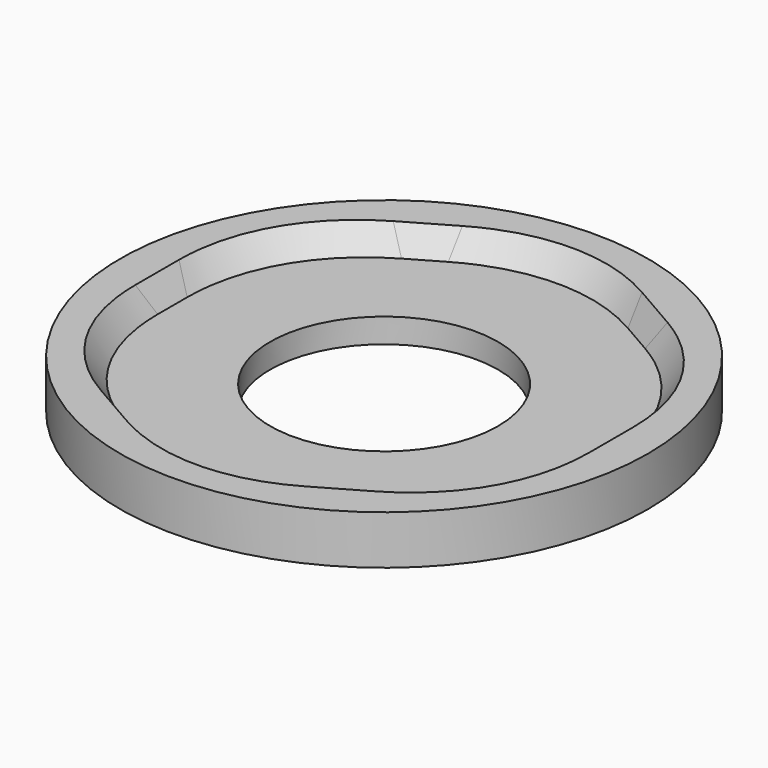
from build123d import *

# Parameters (mm, degrees)
F0_R                   = 32.4
F1_DEPTH               = 6
F0_R_2                 = 14
F2_DEPTH               = 3
F3_DEPTH               = 25
DRAFT_F3_DRAFTED_ANGLE = -32
F4_R                   = 26


# Not quite as in the source:
# - an extrude with a draft is written as a straight extrude whose walls are then drafted


with BuildPart() as f1:
    # F0 (on Top) → F1 (new body)
    with BuildSketch(Plane.XY):
        Circle(F0_R)
        with BuildLine():
            ThreePointArc((25.9807621135, 15), (28.9777747887, 7.7645713531), (30, 0))
            ThreePointArc((30, 0), (28.9777747887, -7.7645713531), (25.9807621135, -15))
            ThreePointArc((25.9807621135, -15), (15, -25.9807621135), (0, -30))
            ThreePointArc((0, -30), (-15, -25.9807621135), (-25.9807621135, -15))
            ThreePointArc((-25.9807621135, -15), (-30, 0), (-25.9807621135, 15))
            ThreePointArc((-25.9807621135, 15), (-15, 25.9807621135), (0, 30))
            ThreePointArc((0, 30), (15, 25.9807621135), (25.9807621135, 15))
        make_face(mode=Mode.SUBTRACT)
        with BuildLine():
            ThreePointArc((0, -30), (15, -25.9807621135), (25.9807621135, -15))
            Line((25.9807621135, -15), (0, -30))
        make_face()
        with BuildLine():
            ThreePointArc((25.9807621135, -15), (28.9777747887, -7.7645713531), (30, 0))
            ThreePointArc((30, 0), (28.9777747887, 7.7645713531), (25.9807621135, 15))
            Line((25.9807621135, 15), (25.9807621135, -15))
        make_face()
        with BuildLine():
            Line((0, 30), (25.9807621135, 15))
            ThreePointArc((25.9807621135, 15), (15, 25.9807621135), (0, 30))
        make_face()
        with BuildLine():
            Line((-25.9807621135, 15), (0, 30))
            ThreePointArc((0, 30), (-15, 25.9807621135), (-25.9807621135, 15))
        make_face()
        with BuildLine():
            Line((-25.9807621135, -15), (-25.9807621135, 15))
            ThreePointArc((-25.9807621135, 15), (-30, 0), (-25.9807621135, -15))
        make_face()
        with BuildLine():
            ThreePointArc((-25.9807621135, -15), (-15, -25.9807621135), (0, -30))
            Line((0, -30), (-25.9807621135, -15))
        make_face()
    extrude(amount=F1_DEPTH)

    # F0 (on Top) → F2 (join)
    with BuildSketch(Plane.XY):
        Polygon((25.9807621135, -15), (25.9807621135, 15), (0, 30), (-25.9807621135, 15), (-25.9807621135, -15), (0, -30), align=None)
        Circle(F0_R_2, mode=Mode.SUBTRACT)
    extrude(amount=F2_DEPTH)


with BuildPart() as f3_drafted:
    # F3 (new): a face of the model
    f3_faces = [f1.part.faces().sort_by_distance(p)[0] for p in [
        (25.1870367202, 0, 3),
    ]]
    extrude(f3_faces, amount=F3_DEPTH)

    # draft_F3_drafted
    draft_f3_drafted_walls = [f3_drafted.faces().sort_by_distance(p)[0] for p in [
        (25.9807621135, 0, 19.6666666667),
        (12.9903810568, 22.5, 19.6666666667),
        (-12.9903810568, 22.5, 19.6666666667),
        (-25.9807621135, 0, 19.6666666667),
        (-12.9903810568, -22.5, 19.6666666667),
        (12.9903810568, -22.5, 19.6666666667),
        (-14, 0, 19.6666666667),
    ]]
    draft(draft_f3_drafted_walls, neutral_plane=Plane.XY.offset(3), angle=DRAFT_F3_DRAFTED_ANGLE)


with BuildPart() as f1_1:
    add(f1.part)

    # join_F3_drafted: cut F3_drafted
    add(f3_drafted.part, mode=Mode.SUBTRACT)

    # F4
    f4_edges = [f1_1.edges().sort_by_distance(p)[0] for p in [
        (26.918066, 15.541153, 4.5),
        (26.918066, -15.541153, 4.5),
        (0, 31.082305, 4.5),
        (-26.918066, 15.541153, 4.5),
        (-26.918066, -15.541153, 4.5),
        (0, -31.082305, 4.5),
    ]]
    fillet(f4_edges, radius=F4_R)


solid = f1_1.part
